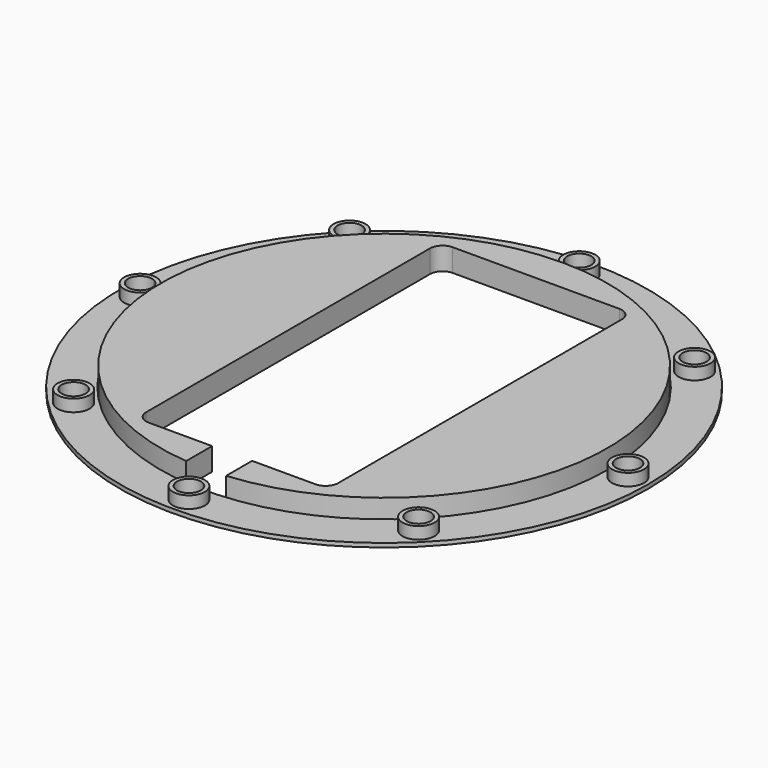
from build123d import *

# Parameters (mm, degrees)
F1_DEPTH = 8.9916
F2_R     = 104.775
F2_R_2   = 4.7625
F2_R_3   = 88.9
F3_DEPTH = 1.5875
F4_R     = 6.35
F4_R_2   = 4.7625
F5_DEPTH = 4.7625


# Not quite as in the source:
# - a feature of the source that left no trace in its solid (it failed there, or was rolled back) is left out
# - the program builds the solid bodies; features that only make, move or delete a surface that nothing else refers to are left out


with BuildPart() as f1:
    # F0 (on Top) → F1 (new body)
    with BuildSketch(Plane.XY):
        with BuildLine():
            ThreePointArc((7.9375, -88.2939329385), (65.4311923894, -59.8128879298), (88.65, 0))
            ThreePointArc((88.65, 0), (-59.8128879298, 65.4311923894), (-7.9375, -88.2939329385))
            Line((-7.9375, -88.2939329385), (-7.9375, -75.40625))
            Line((-7.9375, -75.40625), (-33.1, -75.40625))
            ThreePointArc((-33.1, -75.40625), (-36.6355339059, -73.9417839059), (-38.1, -70.40625))
            Line((-38.1, -70.40625), (-38.1, 70.40625))
            ThreePointArc((-38.1, 70.40625), (-36.6355339059, 73.9417839059), (-33.1, 75.40625))
            Line((-33.1, 75.40625), (33.1, 75.40625))
            ThreePointArc((33.1, 75.40625), (36.6355339059, 73.9417839059), (38.1, 70.40625))
            Line((38.1, 70.40625), (38.1, -70.40625))
            ThreePointArc((38.1, -70.40625), (36.6355339059, -73.9417839059), (33.1, -75.40625))
            Line((33.1, -75.40625), (7.9375, -75.40625))
            Line((7.9375, -75.40625), (7.9375, -88.2939329385))
        make_face()
    extrude(amount=F1_DEPTH)


with BuildPart() as f3:
    # F2 (on Top) → F3 (new body)
    with BuildSketch(Plane.XY):
        Circle(F2_R)
        with Locations((-68.4744529232, -68.4744529232)):
            Circle(F2_R_2, mode=Mode.SUBTRACT)
        with Locations((0, -96.8375)):
            Circle(F2_R_2, mode=Mode.SUBTRACT)
        with Locations((68.4744529232, -68.4744529232)):
            Circle(F2_R_2, mode=Mode.SUBTRACT)
        with Locations((-96.8375, 0)):
            Circle(F2_R_2, mode=Mode.SUBTRACT)
        with Locations((-68.4744529232, 68.4744529232)):
            Circle(F2_R_2, mode=Mode.SUBTRACT)
        Circle(F2_R_3, mode=Mode.SUBTRACT)
        with Locations((96.8375, 0)):
            Circle(F2_R_2, mode=Mode.SUBTRACT)
        with Locations((0, 96.8375)):
            Circle(F2_R_2, mode=Mode.SUBTRACT)
        with Locations((68.4744529232, 68.4744529232)):
            Circle(F2_R_2, mode=Mode.SUBTRACT)
    extrude(amount=F3_DEPTH)

    # F4 (on face) → F5 (join)
    with BuildSketch(Plane.XY.offset(1.5875)):
        with Locations((96.8375, 0)):
            Circle(F4_R)
        with Locations((96.8375, 0)):
            Circle(F4_R_2, mode=Mode.SUBTRACT)
        with Locations((68.4744529232, 68.4744529232)):
            Circle(F4_R)
        with Locations((68.4744529232, 68.4744529232)):
            Circle(F4_R_2, mode=Mode.SUBTRACT)
        with Locations((0, 96.8375)):
            Circle(F4_R)
        with Locations((0, 96.8375)):
            Circle(F4_R_2, mode=Mode.SUBTRACT)
        with Locations((-68.4744529232, 68.4744529232)):
            Circle(F4_R)
        with Locations((-68.4744529232, 68.4744529232)):
            Circle(F4_R_2, mode=Mode.SUBTRACT)
        with Locations((-96.8375, 0)):
            Circle(F4_R)
        with Locations((-96.8375, 0)):
            Circle(F4_R_2, mode=Mode.SUBTRACT)
        with Locations((-68.4744529232, -68.4744529232)):
            Circle(F4_R)
        with Locations((-68.4744529232, -68.4744529232)):
            Circle(F4_R_2, mode=Mode.SUBTRACT)
        with Locations((0, -96.8375)):
            Circle(F4_R)
        with Locations((0, -96.8375)):
            Circle(F4_R_2, mode=Mode.SUBTRACT)
        with Locations((68.4744529232, -68.4744529232)):
            Circle(F4_R)
        with Locations((68.4744529232, -68.4744529232)):
            Circle(F4_R_2, mode=Mode.SUBTRACT)
    extrude(amount=F5_DEPTH)


solid = Compound([f1.part, f3.part])
